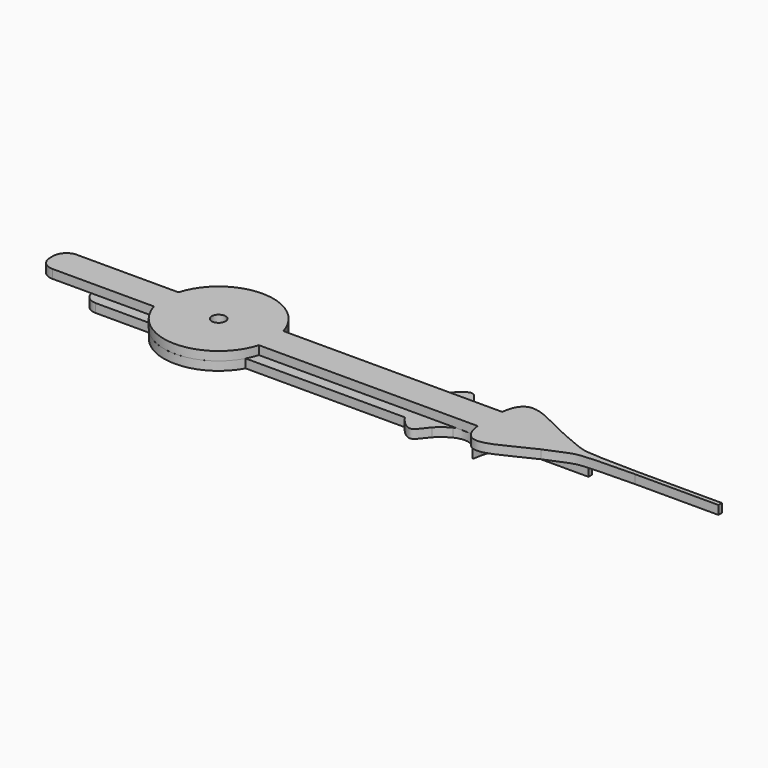
from build123d import *

# Parameters (mm, degrees)
F0_R     = 1.5875
F1_DEPTH = 2
F2_R     = 1.5875
F3_DEPTH = 2
F4_R     = 3
F4_2_R   = 3
F6_DEPTH = 25
F7_R     = 1.5
F8_DEPTH = 25


with BuildPart() as f1:
    # F0 (on Top) → F1 (new body)
    with BuildSketch(Plane.XY):
        with BuildLine():
            ThreePointArc((-12, -3.5), (-12.5, 0), (-12, 3.5))
            Line((-12, 3.5), (-38.25, 3.5))
            Line((-38.25, 3.5), (-38.25, -3.5))
            Line((-38.25, -3.5), (-12, -3.5))
        make_face()
        with BuildLine():
            Line((-12, 3.5), (12, 3.5))
            ThreePointArc((12, 3.5), (0, 12.5), (-12, 3.5))
        make_face()
        with BuildLine():
            Line((62.0709539045, 3.5), (76.5, 3.5))
            add(Edge.make_bspline(
                [(76.5, 3.5), (71.9907153616, 5.4354000871), (64.55282786, 10.6078306891), (62.2970592122, 5.6150011273), (62.0709539045, 3.5)],
                knots=[0, 0, 0, 0, 0.5556190741, 0.8480780717, 0.8480780717, 0.8480780717, 0.8480780717], degree=3))
        make_face()
        with BuildLine():
            Line((12, -3.5), (-12, -3.5))
            ThreePointArc((-12, -3.5), (0, -12.5), (12, -3.5))
        make_face()
        with BuildLine():
            Line((76.5, -3.5), (62.0709539045, -3.5))
            add(Edge.make_bspline(
                [(76.5, -3.5), (71.9907153616, -5.4354000871), (64.55282786, -10.6078306891), (62.2970592122, -5.6150011273), (62.0709539045, -3.5)],
                knots=[0, 0, 0, 0, 0.5556190741, 0.8480780717, 0.8480780717, 0.8480780717, 0.8480780717], degree=3))
        make_face()
        with BuildLine():
            add(Edge.make_bspline(
                [(62.0709539045, 3.5), (61.9535003312, 2.401333), (61.9849445935, 1.196556193), (62.15625, 0)],
                knots=[0.8480780717, 0.8480780717, 0.8480780717, 0.8480780717, 1, 1, 1, 1], degree=3))
            Line((62.0709539045, 3.5), (12, 3.5))
            ThreePointArc((12, 3.5), (12.3743686708, 1.767766953), (12.5, 0))
            ThreePointArc((12.5, 0), (12.3743686708, -1.767766953), (12, -3.5))
            Line((12, -3.5), (62.0709539045, -3.5))
            add(Edge.make_bspline(
                [(62.0709539045, -3.5), (61.9535003312, -2.401333), (61.9849445935, -1.196556193), (62.15625, 0)],
                knots=[0.8480780717, 0.8480780717, 0.8480780717, 0.8480780717, 1, 1, 1, 1], degree=3))
        make_face()
        with BuildLine():
            ThreePointArc((12.5, 0), (12.3743686708, 1.767766953), (12, 3.5))
            Line((12, 3.5), (-12, 3.5))
            ThreePointArc((-12, 3.5), (-12.5, 0), (-12, -3.5))
            Line((-12, -3.5), (12, -3.5))
            ThreePointArc((12, -3.5), (12.3743686708, -1.767766953), (12.5, 0))
        make_face()
        Circle(F0_R, mode=Mode.SUBTRACT)
        with BuildLine():
            add(Edge.make_bspline(
                [(76.5, 3.5), (81.2292632272, 1.3920385639), (83.5245438479, 0.7969108606), (86.4633302777, 0.6546642008), (95.625, 0.5)],
                knots=[0, 0, 0, 0, 0.4354164629, 1, 1, 1, 1], degree=3))
            Line((76.5, 3.5), (62.0709539045, 3.5))
            add(Edge.make_bspline(
                [(62.0709539045, 3.5), (61.9535003312, 2.401333), (61.9849445935, 1.196556193), (62.15625, 0)],
                knots=[0.8480780717, 0.8480780717, 0.8480780717, 0.8480780717, 1, 1, 1, 1], degree=3))
            add(Edge.make_bspline(
                [(62.0709539045, -3.5), (61.9535003312, -2.401333), (61.9849445935, -1.196556193), (62.15625, 0)],
                knots=[0.8480780717, 0.8480780717, 0.8480780717, 0.8480780717, 1, 1, 1, 1], degree=3))
            Line((62.0709539045, -3.5), (76.5, -3.5))
            add(Edge.make_bspline(
                [(76.5, -3.5), (81.2292632272, -1.3920385639), (83.5245438479, -0.7969108606), (86.4633302777, -0.6546642008), (95.625, -0.5)],
                knots=[0, 0, 0, 0, 0.4354164629, 1, 1, 1, 1], degree=3))
            Line((95.625, -0.5), (114.75, -0.5))
            Line((114.75, -0.5), (114.75, 0.5))
            Line((114.75, 0.5), (95.625, 0.5))
        make_face()
    extrude(amount=F1_DEPTH)

    # F4
    f4_edges = [f1.edges().sort_by_distance(p)[0] for p in [
        (-38.25, 3.5, 1),
        (-38.25, -3.5, 1),
    ]]
    fillet(f4_edges, radius=F4_R)


with BuildPart() as f3:
    # F2 (on Top) → F3 (new body)
    with BuildSketch(Plane.XY):
        with BuildLine():
            Line((-10.9658560997, 6), (-26.33333333, 6))
            Line((-26.33333333, 6), (-26.33333333, -6))
            Line((-26.33333333, -6), (-10.9658560997, -6))
            ThreePointArc((-10.9658560997, -6), (-12.5, 0), (-10.9658560997, 6))
        make_face()
        with BuildLine():
            ThreePointArc((10.9658560997, 6), (0, 12.5), (-10.9658560997, 6))
            Line((-10.9658560997, 6), (10.9658560997, 6))
        make_face()
        with BuildLine():
            Line((10.9658560997, -6), (-10.9658560997, -6))
            ThreePointArc((-10.9658560997, -6), (0, -12.5), (10.9658560997, -6))
        make_face()
        with BuildLine():
            Line((53.6581738244, 6), (47.4167542526, 6))
            add(Edge.make_bspline(
                [(47.4167542526, 6), (46.3220957553, 4.3280086445), (45.5684344657, 2.1206918096), (46.0416666667, 0)],
                knots=[0.726906329, 0.726906329, 0.726906329, 0.726906329, 1, 1, 1, 1], degree=3))
            add(Edge.make_bspline(
                [(47.4167542526, -6), (46.3220957553, -4.3280086445), (45.5684344657, -2.1206918096), (46.0416666667, 0)],
                knots=[0.726906329, 0.726906329, 0.726906329, 0.726906329, 1, 1, 1, 1], degree=3))
            Line((47.4167542526, -6), (53.6581738244, -6))
            add(Edge.make_bspline(
                [(56.6666666667, -3.747044364), (55.2992674084, -4.4409490289), (54.3604326541, -5.2428049781), (53.6581738244, -6)],
                knots=[0, 0, 0, 0, 0.1542850544, 0.1542850544, 0.1542850544, 0.1542850544], degree=3))
            add(Edge.make_bspline(
                [(56.6666666667, -3.747044364), (60.0277227864, -2.2489301029), (62.0161168237, -4.2916810168), (63.1679295713, -6)],
                knots=[0, 0, 0, 0, 0.3094476025, 0.3094476025, 0.3094476025, 0.3094476025], degree=3))
            Line((63.1679295713, -6), (64.907909688, -6))
            add(Edge.make_bspline(
                [(64.907909688, -6), (65.3495372223, -3.9292189456), (66.4917594583, -0.8436001546), (70.8333333333, -0.5)],
                knots=[0.6644360976, 0.6644360976, 0.6644360976, 0.6644360976, 1, 1, 1, 1], degree=3))
            Line((70.8333333333, -0.5), (85, -0.5))
            Line((85, -0.5), (85, 0.5))
            Line((85, 0.5), (70.8333333333, 0.5))
            add(Edge.make_bspline(
                [(64.907909688, 6), (65.3495372223, 3.9292189456), (66.4917594583, 0.8436001546), (70.8333333333, 0.5)],
                knots=[0.6644360976, 0.6644360976, 0.6644360976, 0.6644360976, 1, 1, 1, 1], degree=3))
            Line((64.907909688, 6), (63.1679295713, 6))
            add(Edge.make_bspline(
                [(56.6666666667, 3.747044364), (60.0277227864, 2.2489301029), (62.0161168237, 4.2916810168), (63.1679295713, 6)],
                knots=[0, 0, 0, 0, 0.3094476025, 0.3094476025, 0.3094476025, 0.3094476025], degree=3))
            add(Edge.make_bspline(
                [(56.6666666667, 3.747044364), (55.2992674084, 4.4409490289), (54.3604326541, 5.2428049781), (53.6581738244, 6)],
                knots=[0, 0, 0, 0, 0.1542850544, 0.1542850544, 0.1542850544, 0.1542850544], degree=3))
        make_face()
        with BuildLine():
            Line((47.4167542526, 6), (10.9658560997, 6))
            ThreePointArc((10.9658560997, 6), (12.1103922572, 3.0965140685), (12.5, 0))
            ThreePointArc((12.5, 0), (12.1103922572, -3.0965140685), (10.9658560997, -6))
            Line((10.9658560997, -6), (47.4167542526, -6))
            add(Edge.make_bspline(
                [(47.4167542526, -6), (46.3220957553, -4.3280086445), (45.5684344657, -2.1206918096), (46.0416666667, 0)],
                knots=[0.726906329, 0.726906329, 0.726906329, 0.726906329, 1, 1, 1, 1], degree=3))
            add(Edge.make_bspline(
                [(47.4167542526, 6), (46.3220957553, 4.3280086445), (45.5684344657, 2.1206918096), (46.0416666667, 0)],
                knots=[0.726906329, 0.726906329, 0.726906329, 0.726906329, 1, 1, 1, 1], degree=3))
        make_face()
        with BuildLine():
            Line((10.9658560997, 6), (-10.9658560997, 6))
            ThreePointArc((-10.9658560997, 6), (-12.5, 0), (-10.9658560997, -6))
            Line((-10.9658560997, -6), (10.9658560997, -6))
            ThreePointArc((10.9658560997, -6), (12.1103922572, -3.0965140685), (12.5, 0))
            ThreePointArc((12.5, 0), (12.1103922572, 3.0965140685), (10.9658560997, 6))
        make_face()
        Circle(F2_R, mode=Mode.SUBTRACT)
        with BuildLine():
            Line((64.907909688, -6), (63.1679295713, -6))
            add(Edge.make_bspline(
                [(63.1679295713, -6), (63.8278590037, -6.9787788677), (64.5993236597, -8.718696784), (64.6740549365, -7.0965393941), (64.907909688, -6)],
                knots=[0.3094476025, 0.3094476025, 0.3094476025, 0.3094476025, 0.4867451547, 0.6644360976, 0.6644360976, 0.6644360976, 0.6644360976], degree=3))
        make_face()
        with BuildLine():
            add(Edge.make_bspline(
                [(63.1679295713, 6), (63.8278590037, 6.9787788677), (64.5993236597, 8.718696784), (64.6740549365, 7.0965393941), (64.907909688, 6)],
                knots=[0.3094476025, 0.3094476025, 0.3094476025, 0.3094476025, 0.4867451547, 0.6644360976, 0.6644360976, 0.6644360976, 0.6644360976], degree=3))
            Line((63.1679295713, 6), (64.907909688, 6))
        make_face()
        with BuildLine():
            add(Edge.make_bspline(
                [(53.6581738244, 6), (52.2194091826, 7.5513160935), (51.4119093355, 10.0220105563), (48.4450081755, 7.5705644038), (47.4167542526, 6)],
                knots=[0.1542850544, 0.1542850544, 0.1542850544, 0.1542850544, 0.4703791662, 0.726906329, 0.726906329, 0.726906329, 0.726906329], degree=3))
            Line((47.4167542526, 6), (53.6581738244, 6))
        make_face()
        with BuildLine():
            Line((53.6581738244, -6), (47.4167542526, -6))
            add(Edge.make_bspline(
                [(53.6581738244, -6), (52.2194091826, -7.5513160935), (51.4119093355, -10.0220105563), (48.4450081755, -7.5705644038), (47.4167542526, -6)],
                knots=[0.1542850544, 0.1542850544, 0.1542850544, 0.1542850544, 0.4703791662, 0.726906329, 0.726906329, 0.726906329, 0.726906329], degree=3))
        make_face()
    extrude(amount=-F3_DEPTH)

    # F4#2
    f4_2_edges = [f3.edges().sort_by_distance(p)[0] for p in [
        (-26.333333, 6, -1),
        (-26.333333, -6, -1),
    ]]
    fillet(f4_2_edges, radius=F4_2_R)

    # F5 (on face) → F6 (cut)
    with BuildSketch(Plane(origin=(0, 0, -2), x_dir=(1, 0, 0), z_dir=(0, 0, -1))):
        Polygon((44.4125, 0), (50.4125, -3.4641016151), (50.4125, 3.4641016151), align=None)
        Polygon((36.2327160732, -3.5267115138), (38.7950219719, 0), (36.2327160732, 3.5267115138), (32.0868180394, 2.179627584), (32.0868180394, -2.179627584), align=None)
        Polygon((20.3425250947, -3.5355339059), (23.8780590007, 0), (20.3425250947, 3.5355339059), (16.8069911888, 0), align=None)
    extrude(amount=-F6_DEPTH, mode=Mode.SUBTRACT)

    # F7 (on face) → F8 (cut)
    with BuildSketch(Plane(origin=(0, 0, -2), x_dir=(1, 0, 0), z_dir=(0, 0, -1))):
        with Locations((0, 8)):
            Circle(F7_R)
        with Locations((0, -8)):
            Circle(F7_R)
    extrude(amount=-F8_DEPTH, mode=Mode.SUBTRACT)


solid = Compound([f1.part, f3.part])
